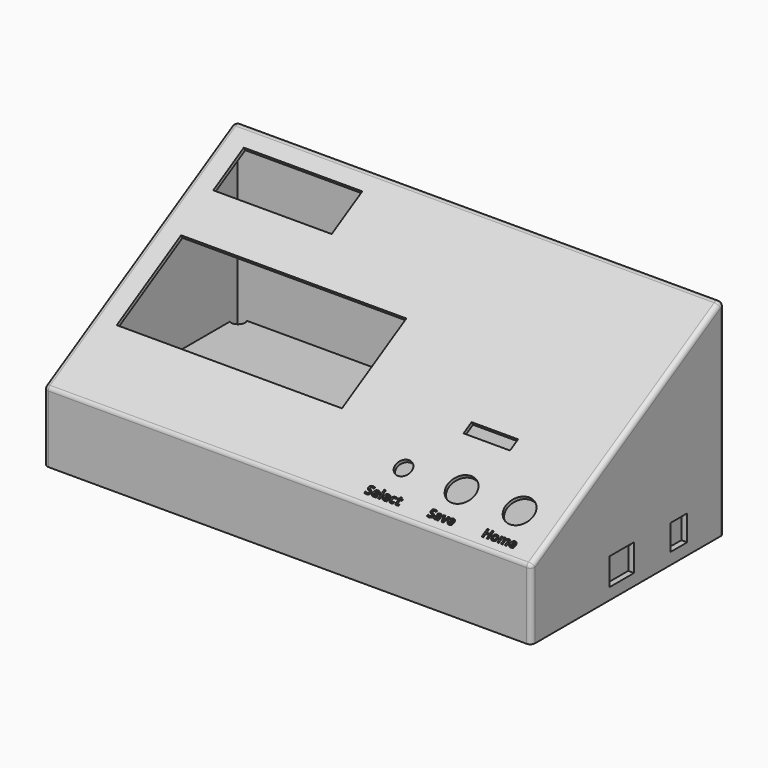
from build123d import *

# Parameters (mm, degrees)
F1_DEPTH       = 210
F2_T           = -1.5
F3_W           = 51
F3_H           = 19
F3_W_2         = 97
F3_H_2         = 40
F3_R           = 3.5
F3_R_2         = 6
F4_DEPTH       = 2.5
F5_W           = 20
F5_H           = 5
F6_DEPTH       = 2.5
F7_TEXT_SIZE   = 4.8611111111
F7_TEXT_SIZE_2 = 5.0900581603
F8_DEPTH       = 1
F9_R           = 2
F10_R          = 3
F11_DEPTH      = 15
F13_DEPTH      = 15
F15_DEPTH      = 15
F16_W          = 9
F16_H          = 11
F16_W_2        = 13.1
F16_H_2        = 11.7
F17_DEPTH      = 2.5
F18_TEXT_SIZE  = 6.9444444444
F19_DEPTH      = 1


# Not quite as in the source:
# - Text() gives the source's letters only with a copy of the font that has no kerning and outlines rounded to 1/6400 em; it was checked with that copy


with BuildPart() as f1:
    # F0 (on Right) → F1 (new body)
    with BuildSketch(Plane.YZ):
        Polygon((0, 30), (0, 0), (103.9230484541, 0), (103.9230484541, 90), align=None)
    extrude(amount=F1_DEPTH)

    # F2
    f2_openings = [f1.faces().sort_by_distance(p)[0] for p in [
        (105, 51.961524, 0),
    ]]
    offset(amount=F2_T, openings=f2_openings)

    # F3 (on face) → F4 (cut)
    with BuildSketch(Plane(origin=(0, -12.9903810568, 22.5), x_dir=(1, 0, 0), z_dir=(0, -0.5, 0.8660254038))):
        with Locations((35.5, 115.5)):
            Rectangle(F3_W, F3_H)
        with Locations((58.5, 66)):
            Rectangle(F3_W_2, F3_H_2)
        with Locations((142.5, 33)):
            Circle(F3_R)
        with Locations((167.5, 33)):
            Circle(F3_R_2)
        with Locations((192.5, 33)):
            Circle(F3_R_2)
    extrude(amount=-F4_DEPTH, mode=Mode.SUBTRACT)

    # F5 (on face) → F6 (cut)
    with BuildSketch(Plane(origin=(0, -12.9903810568, 22.5), x_dir=(1, 0, 0), z_dir=(0, -0.5, 0.8660254038))):
        with Locations((164.5, 55.5)):
            Rectangle(F5_W, F5_H)
    extrude(amount=-F6_DEPTH, mode=Mode.SUBTRACT)

    # F7 (on face) → F8 (cut)
    with BuildSketch(Plane(origin=(0, -12.9903810568, 22.5), x_dir=(1, 0, 0), z_dir=(0, -0.5, 0.8660254038))):
        with Locations((161.9788411458, 19)):
            Text('Save', F7_TEXT_SIZE, font='Open Sans', font_style=FontStyle.BOLD, text_align=(TextAlign.LEFT, TextAlign.BOTTOM))
        with Locations((185.4172092014, 19)):
            Text('Home', F7_TEXT_SIZE, font='Open Sans', font_style=FontStyle.BOLD, text_align=(TextAlign.LEFT, TextAlign.BOTTOM))
        with Locations((134.9830180153, 19)):
            Text('Select', F7_TEXT_SIZE_2, font='Open Sans', font_style=FontStyle.BOLD, text_align=(TextAlign.LEFT, TextAlign.BOTTOM))
    extrude(amount=-F8_DEPTH, mode=Mode.SUBTRACT)

    # F9
    f9_edges = [f1.edges().sort_by_distance(p)[0] for p in [
        (105, 103.923048, 90),
        (210, 51.961524, 60),
        (105, 0, 30),
        (210, 0, 15),
        (0, 51.961524, 60),
        (0, 103.923048, 45),
        (0, 0, 15),
        (210, 103.923048, 45),
    ]]
    fillet(f9_edges, radius=F9_R)

    # F10 (on face) → F11 (join)
    with BuildSketch(Plane(origin=(0, 0, 0), x_dir=(1, 0, 0), z_dir=(0, 0, -1))):
        with Locations((206, -99.9230484541)):
            Circle(F10_R)
    extrude(amount=-F11_DEPTH)

    # F12 (on face) → F13 (join)
    with BuildSketch(Plane(origin=(0, 0, 0), x_dir=(1, 0, 0), z_dir=(0, 0, -1))):
        with BuildLine():
            Line((208.5, -5.6583123952), (208.5, -2.3416876048))
            ThreePointArc((208.5, -2.3416876048), (208.1213203436, -1.8786796564), (207.6583123952, -1.5))
            Line((207.6583123952, -1.5), (204.3416876048, -1.5))
            ThreePointArc((204.3416876048, -1.5), (203.8786796564, -6.1213203436), (208.5, -5.6583123952))
        make_face()
        with BuildLine():
            Line((204.3416876048, -1.5), (207.6583123952, -1.5))
            ThreePointArc((207.6583123952, -1.5), (206, -1), (204.3416876048, -1.5))
        make_face()
    extrude(amount=-F13_DEPTH)

    # F14 (on face) → F15 (join)
    with BuildSketch(Plane(origin=(0, 0, 0), x_dir=(1, 0, 0), z_dir=(0, 0, -1))):
        with BuildLine():
            ThreePointArc((1.5, -98.3249722428), (4.5, -98.3249722428), (6, -100.9230484541))
            ThreePointArc((6, -100.9230484541), (5.8977774789, -101.6995055894), (5.5980762114, -102.4230484541))
            Line((5.5980762114, -102.4230484541), (204.3416876048, -102.4230484541))
            ThreePointArc((204.3416876048, -102.4230484541), (206, -102.9230484541), (207.6583123952, -102.4230484541))
            Line((207.6583123952, -102.4230484541), (208.5, -102.4230484541))
            Line((208.5, -102.4230484541), (208.5, -101.5813608493))
            ThreePointArc((208.5, -101.5813608493), (208.8722813233, -100.7890738579), (209, -99.9230484541))
            ThreePointArc((209, -99.9230484541), (208.8722813233, -99.0570230503), (208.5, -98.264736059))
            Line((208.5, -98.264736059), (208.5, -1.5))
            Line((208.5, -1.5), (5.5980762114, -1.5))
            ThreePointArc((5.5980762114, -1.5), (5.8977774789, -2.2235428647), (6, -3))
            ThreePointArc((6, -3), (4.5, -5.5980762114), (1.5, -5.5980762114))
            Line((1.5, -5.5980762114), (1.5, -98.3249722428))
        make_face()
    extrude(amount=-F15_DEPTH)

    # F16 (on face) → F17 (cut)
    with BuildSketch(Plane.YZ.offset(210)):
        with Locations((79.4230484541, 10.5)):
            Rectangle(F16_W, F16_H)
        with Locations((48.7730484541, 10.85)):
            Rectangle(F16_W_2, F16_H_2)
    extrude(amount=-F17_DEPTH, mode=Mode.SUBTRACT)

    # F18 (on face) → F19 (join)
    with BuildSketch(Plane(origin=(0, 103.9230484541, 0), x_dir=(-1, 0, 0), z_dir=(0, 1, 0))):
        with Locations((-203, 5)):
            Text('Bighead', F18_TEXT_SIZE, font='Open Sans', font_style=FontStyle.BOLD, text_align=(TextAlign.LEFT, TextAlign.BOTTOM))
    extrude(amount=F19_DEPTH)


solid = f1.part
